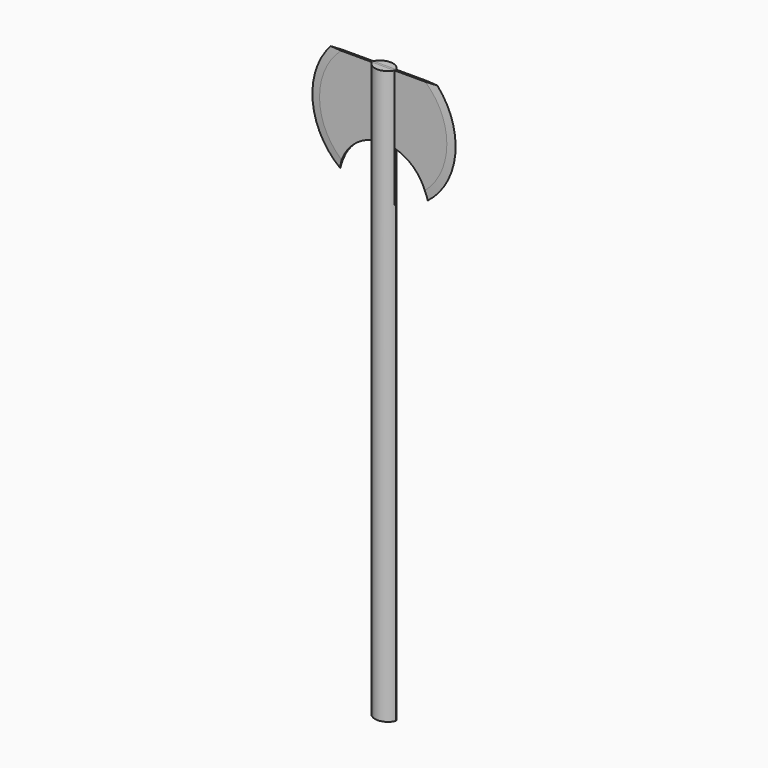
from build123d import *

# Parameters (mm, degrees)
F1_DEPTH      = 914.4
F3_DEPTH      = 1.5875
F3_DEPTH_BACK = 1.5875
F4_SIZE2      = 1.5875
F4_SIZE       = 12.7
F5_SIZE2      = 12.69999
F5_SIZE       = 1.58749
F5_2_SIZE2    = 12.69999
F5_2_SIZE     = 1.58749


# Not quite as in the source:
# - a fillet or chamfer is up to 0.001 mm smaller than in the source, because OpenCascade refuses the exact size


with BuildPart() as f1:
    # F0 (on Top) → F1 (new body)
    with BuildSketch(Plane.XY):
        with BuildLine():
            ThreePointArc((-19.05, 0), (0, -12.7), (19.05, 0))
            ThreePointArc((19.05, 0), (0, 12.7), (-19.05, 0))
        make_face()
    extrude(amount=F1_DEPTH)


with BuildPart() as f3:
    # F2 (on Front) → F3 (new body, two sides)
    with BuildSketch(Plane.XZ) as f3_sk:
        with BuildLine():
            Line((85.1941899427, 914.4), (-85.1941899427, 914.4))
            ThreePointArc((-85.1941899427, 914.4), (-113.8186945704, 827.7217002194), (-69.85, 747.7264265103))
            ThreePointArc((-69.85, 747.7264265103), (-52.7994519478, 783.6641874561), (-19.05, 804.7169389131))
            Line((-19.05, 804.7169389131), (-19.05, 725.498680132))
            ThreePointArc((-19.05, 725.498680132), (0, 723.9), (19.05, 725.498680132))
            Line((19.05, 725.498680132), (19.05, 804.7169389131))
            ThreePointArc((19.05, 804.7169389131), (52.7994519478, 783.6641874561), (69.85, 747.7264265103))
            ThreePointArc((69.85, 747.7264265103), (113.8186945704, 827.7217002194), (85.1941899427, 914.4))
        make_face()
    extrude(amount=F3_DEPTH)
    extrude(f3_sk.sketch, amount=-F3_DEPTH_BACK)

    # F4
    f4_edges = [f3.edges().sort_by_distance(p)[0] for p in [
        (-113.818695, -1.5875, 827.7217),
        (113.818695, -1.5875, 827.7217),
    ]]
    f4_side = f3.faces().sort_by_distance((0, -1.5875, 838.185698))[0]
    chamfer(f4_edges, length=F4_SIZE, length2=F4_SIZE2, reference=f4_side)

    # F5 (size 1.5875 and 12.7 in the source; OpenCascade refuses exactly that, so slightly less here)
    f5_edges = [f3.edges().sort_by_distance(p)[0] for p in [
        (-113.818695, 1.5875, 827.7217),
    ]]
    f5_side = f3.faces().sort_by_distance((-113.818695, 0.79375, 827.7217))[0]
    chamfer(f5_edges, length=F5_SIZE, length2=F5_SIZE2, reference=f5_side)

    # F5#2 (size 1.5875 and 12.7 in the source; OpenCascade refuses exactly that, so slightly less here)
    f5_2_edges = [f3.edges().sort_by_distance(p)[0] for p in [
        (113.818695, 1.5875, 827.7217),
    ]]
    f5_2_side = f3.faces().sort_by_distance((113.818695, 0.79375, 827.7217))[0]
    chamfer(f5_2_edges, length=F5_2_SIZE, length2=F5_2_SIZE2, reference=f5_2_side)


solid = Compound([f1.part, f3.part])
